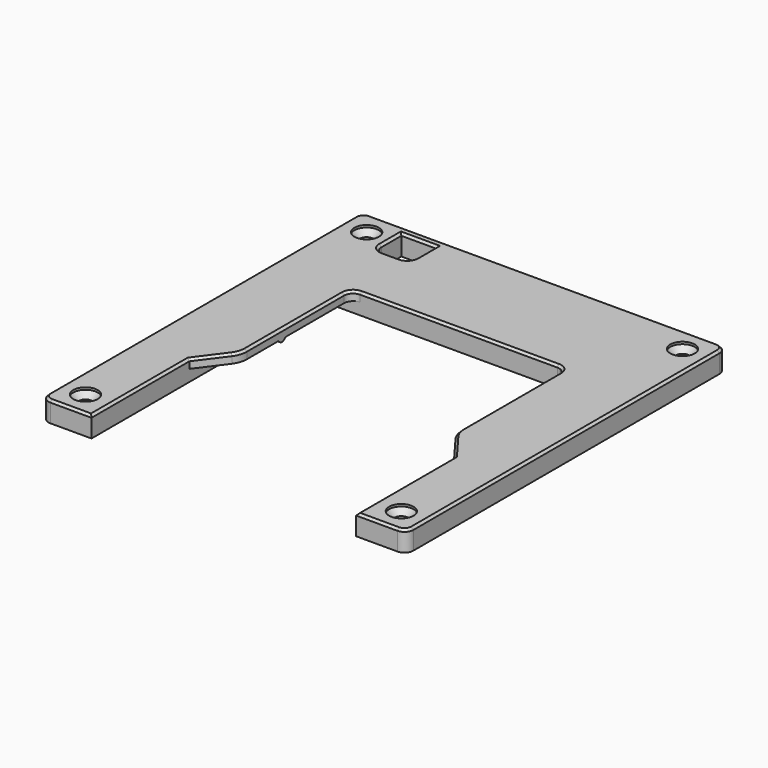
from build123d import *

# Parameters (mm, degrees)
F1_DEPTH      = 2
F3_DEPTH      = 2.2
F5_DEPTH      = 25
F6_R          = 1.5
F7_DEPTH      = 4.2
F8_R          = 2.75
F9_DEPTH      = 2
F10_S5_R      = 1.5
F10_T6_DEPTH  = 5
F10_S11_R     = 1.5
F10_T12_DEPTH = 5
F10_S17_R     = 1.5
F10_T18_DEPTH = 5
F10_S23_R     = 1.5
F10_T24_DEPTH = 5
F11_W         = 5.6
F11_H         = 2
F12_DEPTH     = 0.6
F13_T1_DEPTH  = 8.4722813233
F13_T3_DEPTH  = 8.4722813233
F14_SIZE      = 0.5
F15_DEPTH     = 0.4


# Not quite as in the source:
# - a fillet or chamfer that OpenCascade refuses, or shapes differently, is made with other operations: its cross-section is extruded or revolved along the edge and cut away or added


with BuildPart() as f1:
    # F0 (on Top) → F1 (new body)
    with BuildSketch(Plane.XY):
        with BuildLine():
            Line((80, 0), (2, 0))
            ThreePointArc((2, 0), (0.5857864376, -0.5857864376), (0, -2))
            Line((0, -2), (0, -88))
            ThreePointArc((0, -88), (0.5857864376, -89.4142135624), (2, -90))
            Line((2, -90), (11.25, -90))
            Line((11.25, -90), (11.25, -62.5))
            Line((11.25, -62.5), (15.8564011104, -56.3307127986))
            ThreePointArc((15.8564011104, -56.3307127986), (16.5951030311, -54.9153368199), (16.85, -53.3392666362))
            Line((16.85, -53.3392666362), (16.85, -26))
            ThreePointArc((16.85, -26), (17.4357864376, -24.5857864376), (18.85, -24))
            Line((18.85, -24), (63.15, -24))
            ThreePointArc((63.15, -24), (64.5642135624, -24.5857864376), (65.15, -26))
            Line((65.15, -26), (65.15, -53.3392666362))
            ThreePointArc((65.15, -53.3392666362), (65.4048969689, -54.9153368199), (66.1435988896, -56.3307127986))
            Line((66.1435988896, -56.3307127986), (70.75, -62.5))
            Line((70.75, -62.5), (70.75, -90))
            Line((70.75, -90), (80, -90))
            ThreePointArc((80, -90), (81.4142135624, -89.4142135624), (82, -88))
            Line((82, -88), (82, -2))
            ThreePointArc((82, -2), (81.4142135624, -0.5857864376), (80, 0))
        make_face()
    extrude(amount=F1_DEPTH)

    # F2 (on face) → F3 (join)
    with BuildSketch(Plane(origin=(0, 0, 0), x_dir=(1, 0, 0), z_dir=(0, 0, -1))):
        with BuildLine():
            ThreePointArc((80, 0), (81.4142135624, 0.5857864376), (82, 2))
            Line((82, 2), (82, 88))
            ThreePointArc((82, 88), (81.4142135624, 89.4142135624), (80, 90))
            Line((80, 90), (70.75, 90))
            Line((70.75, 90), (70.75, 62.5))
            Line((70.75, 62.5), (70.75, 26))
            ThreePointArc((70.75, 26), (70.1642135624, 24.5857864376), (68.75, 24))
            Line((68.75, 24), (65.15, 24))
            Line((65.15, 24), (16.85, 24))
            Line((16.85, 24), (13.25, 24))
            ThreePointArc((13.25, 24), (11.8357864376, 24.5857864376), (11.25, 26))
            Line((11.25, 26), (11.25, 62.5))
            Line((11.25, 62.5), (11.25, 90))
            Line((11.25, 90), (2, 90))
            ThreePointArc((2, 90), (0.5857864376, 89.4142135624), (0, 88))
            Line((0, 88), (0, 2))
            ThreePointArc((0, 2), (0.5857864376, 0.5857864376), (2, 0))
            Line((2, 0), (80, 0))
        make_face()
    extrude(amount=F3_DEPTH)

    # F4 (on face) → F5 (cut)
    with BuildSketch(Plane.XY.offset(2)):
        with BuildLine():
            Line((18.3, -2), (10.5, -2))
            Line((10.5, -2), (10.5, -7.6))
            ThreePointArc((10.5, -7.6), (11.0857864376, -9.0142135624), (12.5, -9.6))
            Line((12.5, -9.6), (16.3, -9.6))
            ThreePointArc((16.3, -9.6), (17.7142135624, -9.0142135624), (18.3, -7.6))
            Line((18.3, -7.6), (18.3, -2))
        make_face()
    extrude(amount=-F5_DEPTH, mode=Mode.SUBTRACT)

    # F6 (on face) → F7 (cut)
    with BuildSketch(Plane.XY.offset(2)):
        with Locations((5.5, -84.5)):
            Circle(F6_R)
        with Locations((76.5, -84.5)):
            Circle(F6_R)
        with Locations((5.5, -5.5)):
            Circle(F6_R)
        with Locations((76.5, -5.5)):
            Circle(F6_R)
    extrude(amount=-F7_DEPTH, mode=Mode.SUBTRACT)

    # F8 (on face) → F9 (cut)
    with BuildSketch(Plane.XY.offset(2)):
        with Locations((5.5, -5.5)):
            Circle(F8_R)
        with Locations((76.5, -5.5)):
            Circle(F8_R)
        with Locations((76.5, -84.5)):
            Circle(F8_R)
        with Locations((5.5, -84.5)):
            Circle(F8_R)
    extrude(amount=-F9_DEPTH, mode=Mode.SUBTRACT)

    # F10: chamfer of 1.5 on 4 edges, made by hand


with BuildPart() as f10_tool2:
    # F10_s3 → F10_t4 (revolve)
    with BuildSketch(Plane.XZ.offset(84.5)):
        Polygon((8.25, 1.5), (6.75, 0), (8.25, 0), align=None)
    revolve(axis=Axis((5.5, -84.5, 0), (0, 0, 1)))

    # F10_s5 → F10_t6 (cut, symmetric)
    with BuildSketch(Plane.XY.offset(0.7)):
        with Locations((5.5, -84.5)):
            Circle(F10_S5_R)
    extrude(amount=F10_T6_DEPTH, both=True, mode=Mode.SUBTRACT)


with BuildPart() as f1_1:
    add(f1.part)

    # F10_t1: union F10_tool2
    add(f10_tool2.part)


with BuildPart() as f10_tool8:
    # F10_s9 → F10_t10 (revolve)
    with BuildSketch(Plane.XZ.offset(84.5)):
        Polygon((79.25, 1.5), (77.75, 0), (79.25, 0), align=None)
    revolve(axis=Axis((76.5, -84.5, 0), (0, 0, 1)))

    # F10_s11 → F10_t12 (cut, symmetric)
    with BuildSketch(Plane.XY.offset(0.7)):
        with Locations((76.5, -84.5)):
            Circle(F10_S11_R)
    extrude(amount=F10_T12_DEPTH, both=True, mode=Mode.SUBTRACT)


with BuildPart() as f1_2:
    add(f1_1.part)

    # F10_t7: union F10_tool8
    add(f10_tool8.part)


with BuildPart() as f10_tool14:
    # F10_s15 → F10_t16 (revolve)
    with BuildSketch(Plane.XZ.offset(5.5)):
        Polygon((8.25, 1.5), (6.75, 0), (8.25, 0), align=None)
    revolve(axis=Axis((5.5, -5.5, 0), (0, 0, 1)))

    # F10_s17 → F10_t18 (cut, symmetric)
    with BuildSketch(Plane.XY.offset(0.7)):
        with Locations((5.5, -5.5)):
            Circle(F10_S17_R)
    extrude(amount=F10_T18_DEPTH, both=True, mode=Mode.SUBTRACT)


with BuildPart() as f1_3:
    add(f1_2.part)

    # F10_t13: union F10_tool14
    add(f10_tool14.part)


with BuildPart() as f10_tool20:
    # F10_s21 → F10_t22 (revolve)
    with BuildSketch(Plane.XZ.offset(5.5)):
        Polygon((79.25, 1.5), (77.75, 0), (79.25, 0), align=None)
    revolve(axis=Axis((76.5, -5.5, 0), (0, 0, 1)))

    # F10_s23 → F10_t24 (cut, symmetric)
    with BuildSketch(Plane.XY.offset(0.7)):
        with Locations((76.5, -5.5)):
            Circle(F10_S23_R)
    extrude(amount=F10_T24_DEPTH, both=True, mode=Mode.SUBTRACT)


with BuildPart() as f1_4:
    add(f1_3.part)

    # F10_t19: union F10_tool20
    add(f10_tool20.part)

    # F11 (on face) → F12 (join)
    with BuildSketch(Plane(origin=(0, 0, 0), x_dir=(1, 0, 0), z_dir=(0, 0, -1))):
        with Locations((14.05, 43.5)):
            Rectangle(F11_W, F11_H)
        with Locations((67.95, 43.5)):
            Rectangle(F11_W, F11_H)
    extrude(amount=F12_DEPTH)

    # F13: fillet of radius 1.4 on 4 edges, made by hand

    # F13_s2 → F13_t1 (cut)
    with BuildSketch(Plane.YZ.offset(11.25)):
        with BuildLine():
            ThreePointArc((-42.5, 0), (-43.0008384595, -0.4409673646), (-43.6489125293, -0.6))
            Line((-43.6489125293, -0.6), (-42.5, -0.6))
            Line((-42.5, -0.6), (-42.5, 0))
        make_face()
        with BuildLine():
            ThreePointArc((-43.3510874707, -0.6), (-43.9991615405, -0.4409673646), (-44.5, 0))
            Line((-44.5, 0), (-44.5, -0.6))
            Line((-44.5, -0.6), (-43.3510874707, -0.6))
        make_face()
    extrude(amount=F13_T1_DEPTH, mode=Mode.SUBTRACT)

    # F13_s4 → F13_t3 (cut)
    with BuildSketch(Plane.YZ.offset(62.2777186767)):
        with BuildLine():
            ThreePointArc((-43.6489125293, -0.6), (-43.0008384595, -0.4409673646), (-42.5, 0))
            Line((-42.5, 0), (-42.5, -0.6))
            Line((-42.5, -0.6), (-43.6489125293, -0.6))
        make_face()
        with BuildLine():
            ThreePointArc((-44.5, 0), (-43.9991615405, -0.4409673646), (-43.3510874707, -0.6))
            Line((-43.3510874707, -0.6), (-44.5, -0.6))
            Line((-44.5, -0.6), (-44.5, 0))
        make_face()
    extrude(amount=F13_T3_DEPTH, mode=Mode.SUBTRACT)

    # F14
    f14_edges = [f1_4.edges().sort_by_distance(p)[0] for p in [
        (0.585786, -0.585786, 2),
        (41, 0, 2),
        (0, -45, 2),
        (10.5, -4.8, 2),
        (14.4, -2, 2),
        (18.3, -4.8, 2),
        (17.714214, -9.014214, 2),
        (14.4, -9.6, 2),
        (11.085786, -9.014214, 2),
        (81.414214, -0.585786, 2),
        (82, -45, 2),
        (11.25, -76.25, 2),
        (6.625, -90, 2),
        (0.585786, -89.414214, 2),
        (81.414214, -89.414214, 2),
        (75.375, -90, 2),
        (70.75, -76.25, 2),
        (68.446799, -59.415356, 2),
        (65.404897, -54.915337, 2),
        (65.15, -39.669633, 2),
        (64.564214, -24.585786, 2),
        (41, -24, 2),
        (17.435786, -24.585786, 2),
        (16.85, -39.669633, 2),
        (16.595103, -54.915337, 2),
        (13.553201, -59.415356, 2),
    ]]
    chamfer(f14_edges, length=F14_SIZE)

    # F15 (add): a face of the model
    f15_faces = [f1_4.faces().sort_by_distance(p)[0] for p in [
        (80.5532838324, -1.4467161676, -2.2),
    ]]
    extrude(f15_faces, amount=F15_DEPTH)


solid = f1_4.part
